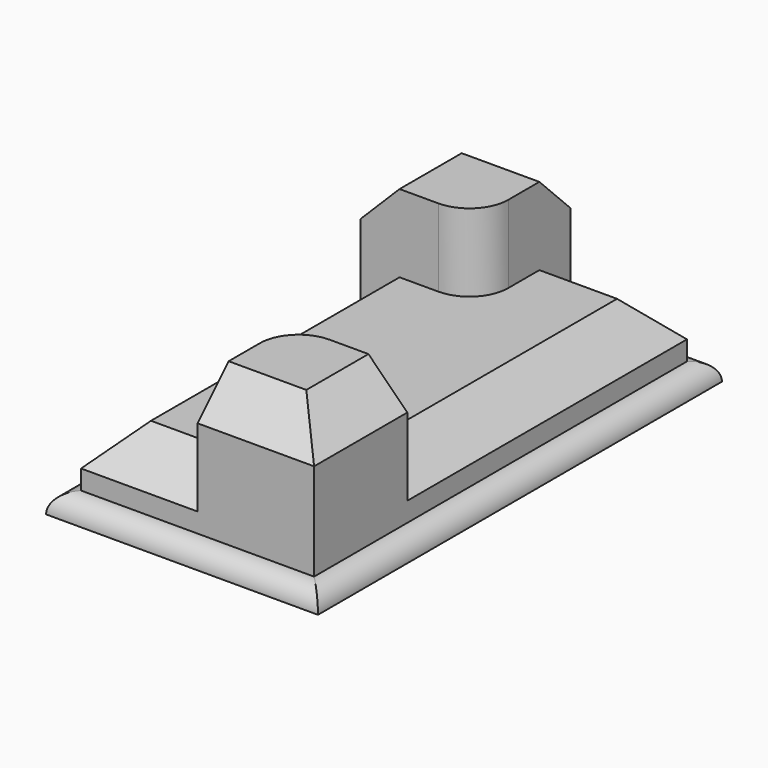
from build123d import *

# Parameters (mm, degrees)
F0_W     = 88.9
F0_H     = 165.1
F1_DEPTH = 6.35
F2_R     = 6.34999
F3_DEPTH = 25.4
F4_SIZE  = 12.7
F5_DEPTH = 50.8
F6_SIZE  = 12.7


# Not quite as in the source:
# - a fillet or chamfer is up to 0.001 mm smaller than in the source, because OpenCascade refuses the exact size


with BuildPart() as f1:
    # F0 (on Top) → F1 (new body)
    with BuildSketch(Plane.XY):
        with Locations((-3.1579616427, 10.7737789035)):
            Rectangle(F0_W, F0_H)
        Polygon((-41.2579616427, 48.8737789035), (-41.2579616427, 86.9737789035), (-3.1579616427, 86.9737789035), (34.9420383573, 86.9737789035), (34.9420383573, -27.3262210965), (34.9420383573, -65.4262210965), (-3.1579616427, -65.4262210965), (-41.2579616427, -65.4262210965), align=None, mode=Mode.SUBTRACT)
    extrude(amount=F1_DEPTH)

    # F2 (radius 6.35 in the source; OpenCascade refuses exactly that, so slightly less here)
    f2_edges = [f1.edges().sort_by_distance(p)[0] for p in [
        (-47.607962, 10.773779, 6.35),
        (-3.157962, 93.323779, 6.35),
        (41.292038, 10.773779, 6.35),
        (-3.157962, -71.776221, 6.35),
    ]]
    fillet(f2_edges, radius=F2_R)

    # F0 (on Top) → F3 (join)
    with BuildSketch(Plane.XY):
        with BuildLine():
            Line((34.9420383573, 86.9737789035), (-3.1579616427, 86.9737789035))
            Line((-3.1579616427, 86.9737789035), (-3.1579616427, 61.5737789035))
            ThreePointArc((-3.1579616427, 61.5737789035), (-6.8777055217, 52.5935227824), (-15.8579616427, 48.8737789035))
            Line((-15.8579616427, 48.8737789035), (-41.2579616427, 48.8737789035))
            Line((-41.2579616427, 48.8737789035), (-41.2579616427, -65.4262210965))
            Line((-41.2579616427, -65.4262210965), (-3.1579616427, -65.4262210965))
            Line((-3.1579616427, -65.4262210965), (-3.1579616427, -40.0262210965))
            ThreePointArc((-3.1579616427, -40.0262210965), (0.5617822362, -31.0459649754), (9.5420383573, -27.3262210965))
            Line((9.5420383573, -27.3262210965), (34.9420383573, -27.3262210965))
            Line((34.9420383573, -27.3262210965), (34.9420383573, 86.9737789035))
        make_face()
    extrude(amount=F3_DEPTH)

    # F4
    f4_edges = [f1.edges().sort_by_distance(p)[0] for p in [
        (34.942038, 29.823779, 25.4),
        (15.892038, 86.973779, 25.4),
        (-41.257962, -8.276221, 25.4),
        (-22.207962, -65.426221, 25.4),
    ]]
    chamfer(f4_edges, length=F4_SIZE)

    # F0 (on Top) → F5 (join)
    with BuildSketch(Plane.XY):
        with BuildLine():
            Line((-3.1579616427, 86.9737789035), (-41.2579616427, 86.9737789035))
            Line((-41.2579616427, 86.9737789035), (-41.2579616427, 48.8737789035))
            Line((-41.2579616427, 48.8737789035), (-15.8579616427, 48.8737789035))
            ThreePointArc((-15.8579616427, 48.8737789035), (-6.8777055217, 52.5935227824), (-3.1579616427, 61.5737789035))
            Line((-3.1579616427, 61.5737789035), (-3.1579616427, 86.9737789035))
        make_face()
        with BuildLine():
            Line((34.9420383573, -65.4262210965), (34.9420383573, -27.3262210965))
            Line((34.9420383573, -27.3262210965), (9.5420383573, -27.3262210965))
            ThreePointArc((9.5420383573, -27.3262210965), (0.5617822362, -31.0459649754), (-3.1579616427, -40.0262210965))
            Line((-3.1579616427, -40.0262210965), (-3.1579616427, -65.4262210965))
            Line((-3.1579616427, -65.4262210965), (34.9420383573, -65.4262210965))
        make_face()
    extrude(amount=F5_DEPTH)

    # F6
    f6_edges = [f1.edges().sort_by_distance(p)[0] for p in [
        (-22.207962, 86.973779, 50.8),
        (-41.257962, 67.923779, 50.8),
        (34.942038, -46.376221, 50.8),
        (15.892038, -65.426221, 50.8),
    ]]
    chamfer(f6_edges, length=F6_SIZE)


solid = f1.part
